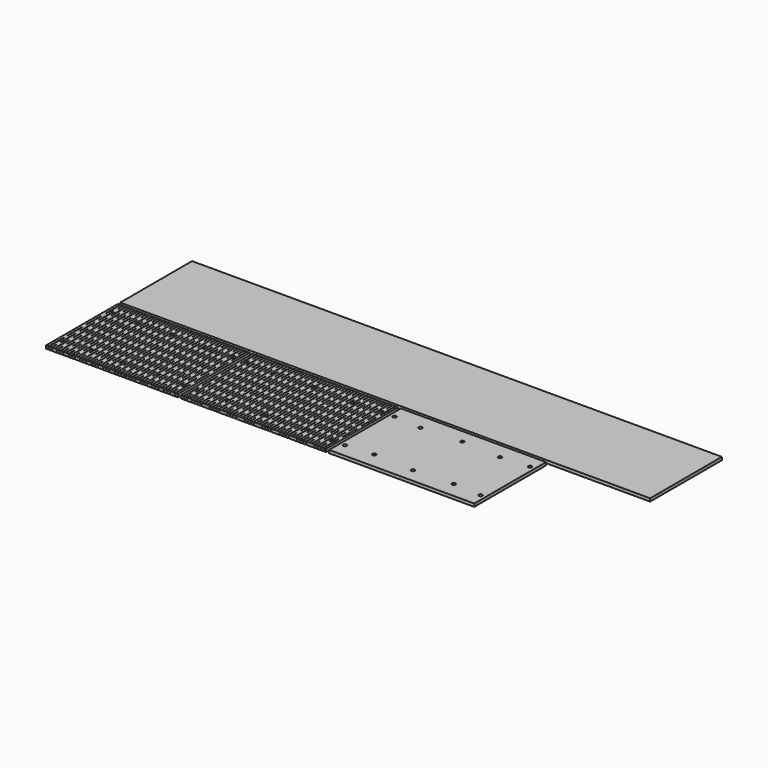
from build123d import *

# Parameters (mm, degrees)
F0_W     = 132.3
F0_H     = 90
F1_DEPTH = 3
F0_W_2   = 531.5
F0_W_3   = 145.6
F2_W     = 0.4
F2_H     = 18.75
F2_H_2   = 6.875
F3_DEPTH = 25
F4_W     = 0.4
F4_H     = 18.75
F4_H_2   = 6.875
F5_DEPTH = 25
F6_D     = 3.5
F6_2_D   = 3.5
F6_3_D   = 3.5
F8_D     = 3.5
F8_2_D   = 3.5
F8_3_D   = 3.5


with BuildPart() as f1:
    # F0 (on Top) → F1 (new body)
    with BuildSketch(Plane.XY):
        with Locations((66.15, -138)):
            Rectangle(F0_W, F0_H)
    extrude(amount=F1_DEPTH)

    # F4 (on face) → F5 (cut)
    with BuildSketch(Plane.XY.offset(3)):
        with Locations((2.7, -173.625)):
            Rectangle(F4_W, F4_H)
        with Locations((5.6, -179.5625)):
            Rectangle(F4_W, F4_H_2)
        with Locations((5.6, -161.75)):
            Rectangle(F4_W, F4_H)
        with Locations((2.7, -149.875)):
            Rectangle(F4_W, F4_H)
        with Locations((5.6, -138)):
            Rectangle(F4_W, F4_H)
        with Locations((2.7, -126.125)):
            Rectangle(F4_W, F4_H)
        with Locations((5.6, -114.25)):
            Rectangle(F4_W, F4_H)
        with Locations((2.7, -102.375)):
            Rectangle(F4_W, F4_H)
        with Locations((5.6, -96.4375)):
            Rectangle(F4_W, F4_H_2)
        with Locations((8.47, -173.625)):
            Rectangle(F4_W, F4_H)
        with Locations((11.37, -179.5625)):
            Rectangle(F4_W, F4_H_2)
        with Locations((11.37, -161.75)):
            Rectangle(F4_W, F4_H)
        with Locations((8.47, -149.875)):
            Rectangle(F4_W, F4_H)
        with Locations((11.37, -138)):
            Rectangle(F4_W, F4_H)
        with Locations((8.47, -126.125)):
            Rectangle(F4_W, F4_H)
        with Locations((11.37, -114.25)):
            Rectangle(F4_W, F4_H)
        with Locations((8.47, -102.375)):
            Rectangle(F4_W, F4_H)
        with Locations((11.37, -96.4375)):
            Rectangle(F4_W, F4_H_2)
        with Locations((14.24, -173.625)):
            Rectangle(F4_W, F4_H)
        with Locations((17.14, -179.5625)):
            Rectangle(F4_W, F4_H_2)
        with Locations((17.14, -161.75)):
            Rectangle(F4_W, F4_H)
        with Locations((14.24, -149.875)):
            Rectangle(F4_W, F4_H)
        with Locations((17.14, -138)):
            Rectangle(F4_W, F4_H)
        with Locations((14.24, -126.125)):
            Rectangle(F4_W, F4_H)
        with Locations((17.14, -114.25)):
            Rectangle(F4_W, F4_H)
        with Locations((14.24, -102.375)):
            Rectangle(F4_W, F4_H)
        with Locations((17.14, -96.4375)):
            Rectangle(F4_W, F4_H_2)
        with Locations((20.01, -173.625)):
            Rectangle(F4_W, F4_H)
        with Locations((22.91, -179.5625)):
            Rectangle(F4_W, F4_H_2)
        with Locations((22.91, -161.75)):
            Rectangle(F4_W, F4_H)
        with Locations((20.01, -149.875)):
            Rectangle(F4_W, F4_H)
        with Locations((22.91, -138)):
            Rectangle(F4_W, F4_H)
        with Locations((20.01, -126.125)):
            Rectangle(F4_W, F4_H)
        with Locations((22.91, -114.25)):
            Rectangle(F4_W, F4_H)
        with Locations((20.01, -102.375)):
            Rectangle(F4_W, F4_H)
        with Locations((22.91, -96.4375)):
            Rectangle(F4_W, F4_H_2)
        with Locations((25.78, -173.625)):
            Rectangle(F4_W, F4_H)
        with Locations((28.68, -179.5625)):
            Rectangle(F4_W, F4_H_2)
        with Locations((28.68, -161.75)):
            Rectangle(F4_W, F4_H)
        with Locations((25.78, -149.875)):
            Rectangle(F4_W, F4_H)
        with Locations((28.68, -138)):
            Rectangle(F4_W, F4_H)
        with Locations((25.78, -126.125)):
            Rectangle(F4_W, F4_H)
        with Locations((28.68, -114.25)):
            Rectangle(F4_W, F4_H)
        with Locations((25.78, -102.375)):
            Rectangle(F4_W, F4_H)
        with Locations((28.68, -96.4375)):
            Rectangle(F4_W, F4_H_2)
        with Locations((31.55, -173.625)):
            Rectangle(F4_W, F4_H)
        with Locations((34.45, -179.5625)):
            Rectangle(F4_W, F4_H_2)
        with Locations((34.45, -161.75)):
            Rectangle(F4_W, F4_H)
        with Locations((31.55, -149.875)):
            Rectangle(F4_W, F4_H)
        with Locations((34.45, -138)):
            Rectangle(F4_W, F4_H)
        with Locations((31.55, -126.125)):
            Rectangle(F4_W, F4_H)
        with Locations((34.45, -114.25)):
            Rectangle(F4_W, F4_H)
        with Locations((31.55, -102.375)):
            Rectangle(F4_W, F4_H)
        with Locations((34.45, -96.4375)):
            Rectangle(F4_W, F4_H_2)
        with Locations((37.32, -173.625)):
            Rectangle(F4_W, F4_H)
        with Locations((40.22, -179.5625)):
            Rectangle(F4_W, F4_H_2)
        with Locations((40.22, -161.75)):
            Rectangle(F4_W, F4_H)
        with Locations((37.32, -149.875)):
            Rectangle(F4_W, F4_H)
        with Locations((40.22, -138)):
            Rectangle(F4_W, F4_H)
        with Locations((37.32, -126.125)):
            Rectangle(F4_W, F4_H)
        with Locations((40.22, -114.25)):
            Rectangle(F4_W, F4_H)
        with Locations((37.32, -102.375)):
            Rectangle(F4_W, F4_H)
        with Locations((40.22, -96.4375)):
            Rectangle(F4_W, F4_H_2)
        with Locations((43.09, -173.625)):
            Rectangle(F4_W, F4_H)
        with Locations((45.99, -179.5625)):
            Rectangle(F4_W, F4_H_2)
        with Locations((45.99, -161.75)):
            Rectangle(F4_W, F4_H)
        with Locations((43.09, -149.875)):
            Rectangle(F4_W, F4_H)
        with Locations((45.99, -138)):
            Rectangle(F4_W, F4_H)
        with Locations((43.09, -126.125)):
            Rectangle(F4_W, F4_H)
        with Locations((45.99, -114.25)):
            Rectangle(F4_W, F4_H)
        with Locations((43.09, -102.375)):
            Rectangle(F4_W, F4_H)
        with Locations((45.99, -96.4375)):
            Rectangle(F4_W, F4_H_2)
        with Locations((48.86, -173.625)):
            Rectangle(F4_W, F4_H)
        with Locations((51.76, -179.5625)):
            Rectangle(F4_W, F4_H_2)
        with Locations((51.76, -161.75)):
            Rectangle(F4_W, F4_H)
        with Locations((48.86, -149.875)):
            Rectangle(F4_W, F4_H)
        with Locations((51.76, -138)):
            Rectangle(F4_W, F4_H)
        with Locations((48.86, -126.125)):
            Rectangle(F4_W, F4_H)
        with Locations((51.76, -114.25)):
            Rectangle(F4_W, F4_H)
        with Locations((48.86, -102.375)):
            Rectangle(F4_W, F4_H)
        with Locations((51.76, -96.4375)):
            Rectangle(F4_W, F4_H_2)
        with Locations((54.63, -173.625)):
            Rectangle(F4_W, F4_H)
        with Locations((57.53, -179.5625)):
            Rectangle(F4_W, F4_H_2)
        with Locations((57.53, -161.75)):
            Rectangle(F4_W, F4_H)
        with Locations((54.63, -149.875)):
            Rectangle(F4_W, F4_H)
        with Locations((57.53, -138)):
            Rectangle(F4_W, F4_H)
        with Locations((54.63, -126.125)):
            Rectangle(F4_W, F4_H)
        with Locations((57.53, -114.25)):
            Rectangle(F4_W, F4_H)
        with Locations((54.63, -102.375)):
            Rectangle(F4_W, F4_H)
        with Locations((57.53, -96.4375)):
            Rectangle(F4_W, F4_H_2)
        with Locations((60.4, -173.625)):
            Rectangle(F4_W, F4_H)
        with Locations((63.3, -179.5625)):
            Rectangle(F4_W, F4_H_2)
        with Locations((63.3, -161.75)):
            Rectangle(F4_W, F4_H)
        with Locations((60.4, -149.875)):
            Rectangle(F4_W, F4_H)
        with Locations((63.3, -138)):
            Rectangle(F4_W, F4_H)
        with Locations((60.4, -126.125)):
            Rectangle(F4_W, F4_H)
        with Locations((63.3, -114.25)):
            Rectangle(F4_W, F4_H)
        with Locations((60.4, -102.375)):
            Rectangle(F4_W, F4_H)
        with Locations((63.3, -96.4375)):
            Rectangle(F4_W, F4_H_2)
        with Locations((66.17, -173.625)):
            Rectangle(F4_W, F4_H)
        with Locations((69.07, -179.5625)):
            Rectangle(F4_W, F4_H_2)
        with Locations((69.07, -161.75)):
            Rectangle(F4_W, F4_H)
        with Locations((66.17, -149.875)):
            Rectangle(F4_W, F4_H)
        with Locations((69.07, -138)):
            Rectangle(F4_W, F4_H)
        with Locations((66.17, -126.125)):
            Rectangle(F4_W, F4_H)
        with Locations((69.07, -114.25)):
            Rectangle(F4_W, F4_H)
        with Locations((66.17, -102.375)):
            Rectangle(F4_W, F4_H)
        with Locations((69.07, -96.4375)):
            Rectangle(F4_W, F4_H_2)
        with Locations((71.94, -173.625)):
            Rectangle(F4_W, F4_H)
        with Locations((74.84, -179.5625)):
            Rectangle(F4_W, F4_H_2)
        with Locations((74.84, -161.75)):
            Rectangle(F4_W, F4_H)
        with Locations((71.94, -149.875)):
            Rectangle(F4_W, F4_H)
        with Locations((74.84, -138)):
            Rectangle(F4_W, F4_H)
        with Locations((71.94, -126.125)):
            Rectangle(F4_W, F4_H)
        with Locations((74.84, -114.25)):
            Rectangle(F4_W, F4_H)
        with Locations((71.94, -102.375)):
            Rectangle(F4_W, F4_H)
        with Locations((74.84, -96.4375)):
            Rectangle(F4_W, F4_H_2)
        with Locations((77.71, -173.625)):
            Rectangle(F4_W, F4_H)
        with Locations((80.61, -179.5625)):
            Rectangle(F4_W, F4_H_2)
        with Locations((80.61, -161.75)):
            Rectangle(F4_W, F4_H)
        with Locations((77.71, -149.875)):
            Rectangle(F4_W, F4_H)
        with Locations((80.61, -138)):
            Rectangle(F4_W, F4_H)
        with Locations((77.71, -126.125)):
            Rectangle(F4_W, F4_H)
        with Locations((80.61, -114.25)):
            Rectangle(F4_W, F4_H)
        with Locations((77.71, -102.375)):
            Rectangle(F4_W, F4_H)
        with Locations((80.61, -96.4375)):
            Rectangle(F4_W, F4_H_2)
        with Locations((83.48, -173.625)):
            Rectangle(F4_W, F4_H)
        with Locations((86.38, -179.5625)):
            Rectangle(F4_W, F4_H_2)
        with Locations((86.38, -161.75)):
            Rectangle(F4_W, F4_H)
        with Locations((83.48, -149.875)):
            Rectangle(F4_W, F4_H)
        with Locations((86.38, -138)):
            Rectangle(F4_W, F4_H)
        with Locations((83.48, -126.125)):
            Rectangle(F4_W, F4_H)
        with Locations((86.38, -114.25)):
            Rectangle(F4_W, F4_H)
        with Locations((83.48, -102.375)):
            Rectangle(F4_W, F4_H)
        with Locations((86.38, -96.4375)):
            Rectangle(F4_W, F4_H_2)
        with Locations((89.25, -173.625)):
            Rectangle(F4_W, F4_H)
        with Locations((92.15, -179.5625)):
            Rectangle(F4_W, F4_H_2)
        with Locations((92.15, -161.75)):
            Rectangle(F4_W, F4_H)
        with Locations((89.25, -149.875)):
            Rectangle(F4_W, F4_H)
        with Locations((92.15, -138)):
            Rectangle(F4_W, F4_H)
        with Locations((89.25, -126.125)):
            Rectangle(F4_W, F4_H)
        with Locations((92.15, -114.25)):
            Rectangle(F4_W, F4_H)
        with Locations((89.25, -102.375)):
            Rectangle(F4_W, F4_H)
        with Locations((92.15, -96.4375)):
            Rectangle(F4_W, F4_H_2)
        with Locations((95.02, -173.625)):
            Rectangle(F4_W, F4_H)
        with Locations((97.92, -179.5625)):
            Rectangle(F4_W, F4_H_2)
        with Locations((97.92, -161.75)):
            Rectangle(F4_W, F4_H)
        with Locations((95.02, -149.875)):
            Rectangle(F4_W, F4_H)
        with Locations((97.92, -138)):
            Rectangle(F4_W, F4_H)
        with Locations((95.02, -126.125)):
            Rectangle(F4_W, F4_H)
        with Locations((97.92, -114.25)):
            Rectangle(F4_W, F4_H)
        with Locations((95.02, -102.375)):
            Rectangle(F4_W, F4_H)
        with Locations((97.92, -96.4375)):
            Rectangle(F4_W, F4_H_2)
        with Locations((100.79, -173.625)):
            Rectangle(F4_W, F4_H)
        with Locations((103.69, -179.5625)):
            Rectangle(F4_W, F4_H_2)
        with Locations((103.69, -161.75)):
            Rectangle(F4_W, F4_H)
        with Locations((100.79, -149.875)):
            Rectangle(F4_W, F4_H)
        with Locations((103.69, -138)):
            Rectangle(F4_W, F4_H)
        with Locations((100.79, -126.125)):
            Rectangle(F4_W, F4_H)
        with Locations((103.69, -114.25)):
            Rectangle(F4_W, F4_H)
        with Locations((100.79, -102.375)):
            Rectangle(F4_W, F4_H)
        with Locations((103.69, -96.4375)):
            Rectangle(F4_W, F4_H_2)
        with Locations((106.56, -173.625)):
            Rectangle(F4_W, F4_H)
        with Locations((109.46, -179.5625)):
            Rectangle(F4_W, F4_H_2)
        with Locations((109.46, -161.75)):
            Rectangle(F4_W, F4_H)
        with Locations((106.56, -149.875)):
            Rectangle(F4_W, F4_H)
        with Locations((109.46, -138)):
            Rectangle(F4_W, F4_H)
        with Locations((106.56, -126.125)):
            Rectangle(F4_W, F4_H)
        with Locations((109.46, -114.25)):
            Rectangle(F4_W, F4_H)
        with Locations((106.56, -102.375)):
            Rectangle(F4_W, F4_H)
        with Locations((109.46, -96.4375)):
            Rectangle(F4_W, F4_H_2)
        with Locations((112.33, -173.625)):
            Rectangle(F4_W, F4_H)
        with Locations((115.23, -179.5625)):
            Rectangle(F4_W, F4_H_2)
        with Locations((115.23, -161.75)):
            Rectangle(F4_W, F4_H)
        with Locations((112.33, -149.875)):
            Rectangle(F4_W, F4_H)
        with Locations((115.23, -138)):
            Rectangle(F4_W, F4_H)
        with Locations((112.33, -126.125)):
            Rectangle(F4_W, F4_H)
        with Locations((115.23, -114.25)):
            Rectangle(F4_W, F4_H)
        with Locations((112.33, -102.375)):
            Rectangle(F4_W, F4_H)
        with Locations((115.23, -96.4375)):
            Rectangle(F4_W, F4_H_2)
        with Locations((118.1, -173.625)):
            Rectangle(F4_W, F4_H)
        with Locations((121, -179.5625)):
            Rectangle(F4_W, F4_H_2)
        with Locations((121, -161.75)):
            Rectangle(F4_W, F4_H)
        with Locations((118.1, -149.875)):
            Rectangle(F4_W, F4_H)
        with Locations((121, -138)):
            Rectangle(F4_W, F4_H)
        with Locations((118.1, -126.125)):
            Rectangle(F4_W, F4_H)
        with Locations((121, -114.25)):
            Rectangle(F4_W, F4_H)
        with Locations((118.1, -102.375)):
            Rectangle(F4_W, F4_H)
        with Locations((121, -96.4375)):
            Rectangle(F4_W, F4_H_2)
        with Locations((123.87, -173.625)):
            Rectangle(F4_W, F4_H)
        with Locations((126.77, -179.5625)):
            Rectangle(F4_W, F4_H_2)
        with Locations((126.77, -161.75)):
            Rectangle(F4_W, F4_H)
        with Locations((123.87, -149.875)):
            Rectangle(F4_W, F4_H)
        with Locations((126.77, -138)):
            Rectangle(F4_W, F4_H)
        with Locations((123.87, -126.125)):
            Rectangle(F4_W, F4_H)
        with Locations((126.77, -114.25)):
            Rectangle(F4_W, F4_H)
        with Locations((123.87, -102.375)):
            Rectangle(F4_W, F4_H)
        with Locations((126.77, -96.4375)):
            Rectangle(F4_W, F4_H_2)
        with Locations((129.64, -173.625)):
            Rectangle(F4_W, F4_H)
        with Locations((132.54, -179.5625)):
            Rectangle(F4_W, F4_H_2)
        with Locations((132.54, -161.75)):
            Rectangle(F4_W, F4_H)
        with Locations((129.64, -149.875)):
            Rectangle(F4_W, F4_H)
        with Locations((132.54, -138)):
            Rectangle(F4_W, F4_H)
        with Locations((129.64, -126.125)):
            Rectangle(F4_W, F4_H)
        with Locations((132.54, -114.25)):
            Rectangle(F4_W, F4_H)
        with Locations((129.64, -102.375)):
            Rectangle(F4_W, F4_H)
        with Locations((132.54, -96.4375)):
            Rectangle(F4_W, F4_H_2)
    extrude(amount=-F5_DEPTH, mode=Mode.SUBTRACT)

    # F6 (through all)
    with Locations(Plane(origin=(0, 0, 0), x_dir=(1, 0, 0), z_dir=(0, 0, -1))):
        with Locations((32.85, 109), (99.45, 109), (32.85, 167), (99.45, 167), (168.65, 109), (168.65, 167), (248.55, 109), (248.55, 167), (316.25, 109), (396.15, 109), (396.15, 167), (316.25, 167)):
            Hole(F6_D / 2)

    # F8 (through all)
    with Locations(Plane.XY.offset(3)):
        with Locations((4.9, -107), (4.9, -169), (127.4, -107), (127.4, -169), (140.2, -107), (140.2, -169), (276, -169), (276, -107), (288.8, -107), (288.8, -169), (424.6, -107), (424.6, -169), (66.15, -107), (66.15, -169), (208.1, -107), (208.1, -169), (356.7, -107), (356.7, -169)):
            Hole(F8_D / 2)


with BuildPart() as f1b:
    # F0 (on Top) → F1, piece 2 (new body)
    with BuildSketch(Plane.XY):
        with Locations((265.75, -45)):
            Rectangle(F0_W_2, F0_H)
    extrude(amount=F1_DEPTH)


with BuildPart() as f1c:
    # F0 (on Top) → F1, piece 3 (new body)
    with BuildSketch(Plane.XY):
        with Locations((208.1, -138)):
            Rectangle(F0_W_3, F0_H)
    extrude(amount=F1_DEPTH)

    # F2 (on face) → F3 (cut)
    with BuildSketch(Plane.XY.offset(3)):
        with Locations((138, -173.625)):
            Rectangle(F2_W, F2_H)
        with Locations((140.9, -179.5625)):
            Rectangle(F2_W, F2_H_2)
        with Locations((140.9, -161.75)):
            Rectangle(F2_W, F2_H)
        with Locations((138, -149.875)):
            Rectangle(F2_W, F2_H)
        with Locations((140.9, -138)):
            Rectangle(F2_W, F2_H)
        with Locations((138, -126.125)):
            Rectangle(F2_W, F2_H)
        with Locations((140.9, -114.25)):
            Rectangle(F2_W, F2_H)
        with Locations((138, -102.375)):
            Rectangle(F2_W, F2_H)
        with Locations((140.9, -96.4375)):
            Rectangle(F2_W, F2_H_2)
        with Locations((146.75, -96.4375)):
            Rectangle(F2_W, F2_H_2)
        with Locations((146.75, -161.75)):
            Rectangle(F2_W, F2_H)
        with Locations((146.75, -114.25)):
            Rectangle(F2_W, F2_H)
        with Locations((143.85, -149.875)):
            Rectangle(F2_W, F2_H)
        with Locations((146.75, -138)):
            Rectangle(F2_W, F2_H)
        with Locations((143.85, -173.625)):
            Rectangle(F2_W, F2_H)
        with Locations((146.75, -179.5625)):
            Rectangle(F2_W, F2_H_2)
        with Locations((143.85, -126.125)):
            Rectangle(F2_W, F2_H)
        with Locations((143.85, -102.375)):
            Rectangle(F2_W, F2_H)
        with Locations((152.6, -96.4375)):
            Rectangle(F2_W, F2_H_2)
        with Locations((152.6, -161.75)):
            Rectangle(F2_W, F2_H)
        with Locations((152.6, -114.25)):
            Rectangle(F2_W, F2_H)
        with Locations((149.7, -149.875)):
            Rectangle(F2_W, F2_H)
        with Locations((152.6, -138)):
            Rectangle(F2_W, F2_H)
        with Locations((149.7, -173.625)):
            Rectangle(F2_W, F2_H)
        with Locations((152.6, -179.5625)):
            Rectangle(F2_W, F2_H_2)
        with Locations((149.7, -126.125)):
            Rectangle(F2_W, F2_H)
        with Locations((149.7, -102.375)):
            Rectangle(F2_W, F2_H)
        with Locations((158.45, -96.4375)):
            Rectangle(F2_W, F2_H_2)
        with Locations((158.45, -161.75)):
            Rectangle(F2_W, F2_H)
        with Locations((158.45, -114.25)):
            Rectangle(F2_W, F2_H)
        with Locations((155.55, -149.875)):
            Rectangle(F2_W, F2_H)
        with Locations((158.45, -138)):
            Rectangle(F2_W, F2_H)
        with Locations((155.55, -173.625)):
            Rectangle(F2_W, F2_H)
        with Locations((158.45, -179.5625)):
            Rectangle(F2_W, F2_H_2)
        with Locations((155.55, -126.125)):
            Rectangle(F2_W, F2_H)
        with Locations((155.55, -102.375)):
            Rectangle(F2_W, F2_H)
        with Locations((164.3, -96.4375)):
            Rectangle(F2_W, F2_H_2)
        with Locations((164.3, -161.75)):
            Rectangle(F2_W, F2_H)
        with Locations((164.3, -114.25)):
            Rectangle(F2_W, F2_H)
        with Locations((161.4, -149.875)):
            Rectangle(F2_W, F2_H)
        with Locations((164.3, -138)):
            Rectangle(F2_W, F2_H)
        with Locations((161.4, -173.625)):
            Rectangle(F2_W, F2_H)
        with Locations((164.3, -179.5625)):
            Rectangle(F2_W, F2_H_2)
        with Locations((161.4, -126.125)):
            Rectangle(F2_W, F2_H)
        with Locations((161.4, -102.375)):
            Rectangle(F2_W, F2_H)
        with Locations((170.15, -96.4375)):
            Rectangle(F2_W, F2_H_2)
        with Locations((170.15, -161.75)):
            Rectangle(F2_W, F2_H)
        with Locations((170.15, -114.25)):
            Rectangle(F2_W, F2_H)
        with Locations((167.25, -149.875)):
            Rectangle(F2_W, F2_H)
        with Locations((170.15, -138)):
            Rectangle(F2_W, F2_H)
        with Locations((167.25, -173.625)):
            Rectangle(F2_W, F2_H)
        with Locations((170.15, -179.5625)):
            Rectangle(F2_W, F2_H_2)
        with Locations((167.25, -126.125)):
            Rectangle(F2_W, F2_H)
        with Locations((167.25, -102.375)):
            Rectangle(F2_W, F2_H)
        with Locations((176, -96.4375)):
            Rectangle(F2_W, F2_H_2)
        with Locations((176, -161.75)):
            Rectangle(F2_W, F2_H)
        with Locations((176, -114.25)):
            Rectangle(F2_W, F2_H)
        with Locations((173.1, -149.875)):
            Rectangle(F2_W, F2_H)
        with Locations((176, -138)):
            Rectangle(F2_W, F2_H)
        with Locations((173.1, -173.625)):
            Rectangle(F2_W, F2_H)
        with Locations((176, -179.5625)):
            Rectangle(F2_W, F2_H_2)
        with Locations((173.1, -126.125)):
            Rectangle(F2_W, F2_H)
        with Locations((173.1, -102.375)):
            Rectangle(F2_W, F2_H)
        with Locations((181.85, -96.4375)):
            Rectangle(F2_W, F2_H_2)
        with Locations((181.85, -161.75)):
            Rectangle(F2_W, F2_H)
        with Locations((181.85, -114.25)):
            Rectangle(F2_W, F2_H)
        with Locations((178.95, -149.875)):
            Rectangle(F2_W, F2_H)
        with Locations((181.85, -138)):
            Rectangle(F2_W, F2_H)
        with Locations((178.95, -173.625)):
            Rectangle(F2_W, F2_H)
        with Locations((181.85, -179.5625)):
            Rectangle(F2_W, F2_H_2)
        with Locations((178.95, -126.125)):
            Rectangle(F2_W, F2_H)
        with Locations((178.95, -102.375)):
            Rectangle(F2_W, F2_H)
        with Locations((187.7, -96.4375)):
            Rectangle(F2_W, F2_H_2)
        with Locations((187.7, -161.75)):
            Rectangle(F2_W, F2_H)
        with Locations((187.7, -114.25)):
            Rectangle(F2_W, F2_H)
        with Locations((184.8, -149.875)):
            Rectangle(F2_W, F2_H)
        with Locations((187.7, -138)):
            Rectangle(F2_W, F2_H)
        with Locations((184.8, -173.625)):
            Rectangle(F2_W, F2_H)
        with Locations((187.7, -179.5625)):
            Rectangle(F2_W, F2_H_2)
        with Locations((184.8, -126.125)):
            Rectangle(F2_W, F2_H)
        with Locations((184.8, -102.375)):
            Rectangle(F2_W, F2_H)
        with Locations((193.55, -96.4375)):
            Rectangle(F2_W, F2_H_2)
        with Locations((193.55, -161.75)):
            Rectangle(F2_W, F2_H)
        with Locations((193.55, -114.25)):
            Rectangle(F2_W, F2_H)
        with Locations((190.65, -149.875)):
            Rectangle(F2_W, F2_H)
        with Locations((193.55, -138)):
            Rectangle(F2_W, F2_H)
        with Locations((190.65, -173.625)):
            Rectangle(F2_W, F2_H)
        with Locations((193.55, -179.5625)):
            Rectangle(F2_W, F2_H_2)
        with Locations((190.65, -126.125)):
            Rectangle(F2_W, F2_H)
        with Locations((190.65, -102.375)):
            Rectangle(F2_W, F2_H)
        with Locations((199.4, -96.4375)):
            Rectangle(F2_W, F2_H_2)
        with Locations((199.4, -161.75)):
            Rectangle(F2_W, F2_H)
        with Locations((199.4, -114.25)):
            Rectangle(F2_W, F2_H)
        with Locations((196.5, -149.875)):
            Rectangle(F2_W, F2_H)
        with Locations((199.4, -138)):
            Rectangle(F2_W, F2_H)
        with Locations((196.5, -173.625)):
            Rectangle(F2_W, F2_H)
        with Locations((199.4, -179.5625)):
            Rectangle(F2_W, F2_H_2)
        with Locations((196.5, -126.125)):
            Rectangle(F2_W, F2_H)
        with Locations((196.5, -102.375)):
            Rectangle(F2_W, F2_H)
        with Locations((205.25, -96.4375)):
            Rectangle(F2_W, F2_H_2)
        with Locations((205.25, -161.75)):
            Rectangle(F2_W, F2_H)
        with Locations((205.25, -114.25)):
            Rectangle(F2_W, F2_H)
        with Locations((202.35, -149.875)):
            Rectangle(F2_W, F2_H)
        with Locations((205.25, -138)):
            Rectangle(F2_W, F2_H)
        with Locations((202.35, -173.625)):
            Rectangle(F2_W, F2_H)
        with Locations((205.25, -179.5625)):
            Rectangle(F2_W, F2_H_2)
        with Locations((202.35, -126.125)):
            Rectangle(F2_W, F2_H)
        with Locations((202.35, -102.375)):
            Rectangle(F2_W, F2_H)
        with Locations((211.1, -96.4375)):
            Rectangle(F2_W, F2_H_2)
        with Locations((211.1, -161.75)):
            Rectangle(F2_W, F2_H)
        with Locations((211.1, -114.25)):
            Rectangle(F2_W, F2_H)
        with Locations((208.2, -149.875)):
            Rectangle(F2_W, F2_H)
        with Locations((211.1, -138)):
            Rectangle(F2_W, F2_H)
        with Locations((208.2, -173.625)):
            Rectangle(F2_W, F2_H)
        with Locations((211.1, -179.5625)):
            Rectangle(F2_W, F2_H_2)
        with Locations((208.2, -126.125)):
            Rectangle(F2_W, F2_H)
        with Locations((208.2, -102.375)):
            Rectangle(F2_W, F2_H)
        with Locations((216.95, -96.4375)):
            Rectangle(F2_W, F2_H_2)
        with Locations((216.95, -161.75)):
            Rectangle(F2_W, F2_H)
        with Locations((216.95, -114.25)):
            Rectangle(F2_W, F2_H)
        with Locations((214.05, -149.875)):
            Rectangle(F2_W, F2_H)
        with Locations((216.95, -138)):
            Rectangle(F2_W, F2_H)
        with Locations((214.05, -173.625)):
            Rectangle(F2_W, F2_H)
        with Locations((216.95, -179.5625)):
            Rectangle(F2_W, F2_H_2)
        with Locations((214.05, -126.125)):
            Rectangle(F2_W, F2_H)
        with Locations((214.05, -102.375)):
            Rectangle(F2_W, F2_H)
        with Locations((222.8, -96.4375)):
            Rectangle(F2_W, F2_H_2)
        with Locations((222.8, -161.75)):
            Rectangle(F2_W, F2_H)
        with Locations((222.8, -114.25)):
            Rectangle(F2_W, F2_H)
        with Locations((219.9, -149.875)):
            Rectangle(F2_W, F2_H)
        with Locations((222.8, -138)):
            Rectangle(F2_W, F2_H)
        with Locations((219.9, -173.625)):
            Rectangle(F2_W, F2_H)
        with Locations((222.8, -179.5625)):
            Rectangle(F2_W, F2_H_2)
        with Locations((219.9, -126.125)):
            Rectangle(F2_W, F2_H)
        with Locations((219.9, -102.375)):
            Rectangle(F2_W, F2_H)
        with Locations((228.65, -96.4375)):
            Rectangle(F2_W, F2_H_2)
        with Locations((228.65, -161.75)):
            Rectangle(F2_W, F2_H)
        with Locations((228.65, -114.25)):
            Rectangle(F2_W, F2_H)
        with Locations((225.75, -149.875)):
            Rectangle(F2_W, F2_H)
        with Locations((228.65, -138)):
            Rectangle(F2_W, F2_H)
        with Locations((225.75, -173.625)):
            Rectangle(F2_W, F2_H)
        with Locations((228.65, -179.5625)):
            Rectangle(F2_W, F2_H_2)
        with Locations((225.75, -126.125)):
            Rectangle(F2_W, F2_H)
        with Locations((225.75, -102.375)):
            Rectangle(F2_W, F2_H)
        with Locations((234.5, -96.4375)):
            Rectangle(F2_W, F2_H_2)
        with Locations((234.5, -161.75)):
            Rectangle(F2_W, F2_H)
        with Locations((234.5, -114.25)):
            Rectangle(F2_W, F2_H)
        with Locations((231.6, -149.875)):
            Rectangle(F2_W, F2_H)
        with Locations((234.5, -138)):
            Rectangle(F2_W, F2_H)
        with Locations((231.6, -173.625)):
            Rectangle(F2_W, F2_H)
        with Locations((234.5, -179.5625)):
            Rectangle(F2_W, F2_H_2)
        with Locations((231.6, -126.125)):
            Rectangle(F2_W, F2_H)
        with Locations((231.6, -102.375)):
            Rectangle(F2_W, F2_H)
        with Locations((240.35, -96.4375)):
            Rectangle(F2_W, F2_H_2)
        with Locations((240.35, -161.75)):
            Rectangle(F2_W, F2_H)
        with Locations((240.35, -114.25)):
            Rectangle(F2_W, F2_H)
        with Locations((237.45, -149.875)):
            Rectangle(F2_W, F2_H)
        with Locations((240.35, -138)):
            Rectangle(F2_W, F2_H)
        with Locations((237.45, -173.625)):
            Rectangle(F2_W, F2_H)
        with Locations((240.35, -179.5625)):
            Rectangle(F2_W, F2_H_2)
        with Locations((237.45, -126.125)):
            Rectangle(F2_W, F2_H)
        with Locations((237.45, -102.375)):
            Rectangle(F2_W, F2_H)
        with Locations((246.2, -96.4375)):
            Rectangle(F2_W, F2_H_2)
        with Locations((246.2, -161.75)):
            Rectangle(F2_W, F2_H)
        with Locations((246.2, -114.25)):
            Rectangle(F2_W, F2_H)
        with Locations((243.3, -149.875)):
            Rectangle(F2_W, F2_H)
        with Locations((246.2, -138)):
            Rectangle(F2_W, F2_H)
        with Locations((243.3, -173.625)):
            Rectangle(F2_W, F2_H)
        with Locations((246.2, -179.5625)):
            Rectangle(F2_W, F2_H_2)
        with Locations((243.3, -126.125)):
            Rectangle(F2_W, F2_H)
        with Locations((243.3, -102.375)):
            Rectangle(F2_W, F2_H)
        with Locations((252.05, -96.4375)):
            Rectangle(F2_W, F2_H_2)
        with Locations((252.05, -161.75)):
            Rectangle(F2_W, F2_H)
        with Locations((252.05, -114.25)):
            Rectangle(F2_W, F2_H)
        with Locations((249.15, -149.875)):
            Rectangle(F2_W, F2_H)
        with Locations((252.05, -138)):
            Rectangle(F2_W, F2_H)
        with Locations((249.15, -173.625)):
            Rectangle(F2_W, F2_H)
        with Locations((252.05, -179.5625)):
            Rectangle(F2_W, F2_H_2)
        with Locations((249.15, -126.125)):
            Rectangle(F2_W, F2_H)
        with Locations((249.15, -102.375)):
            Rectangle(F2_W, F2_H)
        with Locations((257.9, -96.4375)):
            Rectangle(F2_W, F2_H_2)
        with Locations((257.9, -161.75)):
            Rectangle(F2_W, F2_H)
        with Locations((257.9, -114.25)):
            Rectangle(F2_W, F2_H)
        with Locations((255, -149.875)):
            Rectangle(F2_W, F2_H)
        with Locations((257.9, -138)):
            Rectangle(F2_W, F2_H)
        with Locations((255, -173.625)):
            Rectangle(F2_W, F2_H)
        with Locations((257.9, -179.5625)):
            Rectangle(F2_W, F2_H_2)
        with Locations((255, -126.125)):
            Rectangle(F2_W, F2_H)
        with Locations((255, -102.375)):
            Rectangle(F2_W, F2_H)
        with Locations((263.75, -96.4375)):
            Rectangle(F2_W, F2_H_2)
        with Locations((263.75, -161.75)):
            Rectangle(F2_W, F2_H)
        with Locations((263.75, -114.25)):
            Rectangle(F2_W, F2_H)
        with Locations((260.85, -149.875)):
            Rectangle(F2_W, F2_H)
        with Locations((263.75, -138)):
            Rectangle(F2_W, F2_H)
        with Locations((260.85, -173.625)):
            Rectangle(F2_W, F2_H)
        with Locations((263.75, -179.5625)):
            Rectangle(F2_W, F2_H_2)
        with Locations((260.85, -126.125)):
            Rectangle(F2_W, F2_H)
        with Locations((260.85, -102.375)):
            Rectangle(F2_W, F2_H)
        with Locations((269.6, -96.4375)):
            Rectangle(F2_W, F2_H_2)
        with Locations((269.6, -161.75)):
            Rectangle(F2_W, F2_H)
        with Locations((269.6, -114.25)):
            Rectangle(F2_W, F2_H)
        with Locations((266.7, -149.875)):
            Rectangle(F2_W, F2_H)
        with Locations((269.6, -138)):
            Rectangle(F2_W, F2_H)
        with Locations((266.7, -173.625)):
            Rectangle(F2_W, F2_H)
        with Locations((269.6, -179.5625)):
            Rectangle(F2_W, F2_H_2)
        with Locations((266.7, -126.125)):
            Rectangle(F2_W, F2_H)
        with Locations((266.7, -102.375)):
            Rectangle(F2_W, F2_H)
        with Locations((275.45, -96.4375)):
            Rectangle(F2_W, F2_H_2)
        with Locations((275.45, -161.75)):
            Rectangle(F2_W, F2_H)
        with Locations((275.45, -114.25)):
            Rectangle(F2_W, F2_H)
        with Locations((272.55, -149.875)):
            Rectangle(F2_W, F2_H)
        with Locations((275.45, -138)):
            Rectangle(F2_W, F2_H)
        with Locations((272.55, -173.625)):
            Rectangle(F2_W, F2_H)
        with Locations((275.45, -179.5625)):
            Rectangle(F2_W, F2_H_2)
        with Locations((272.55, -126.125)):
            Rectangle(F2_W, F2_H)
        with Locations((272.55, -102.375)):
            Rectangle(F2_W, F2_H)
        with Locations((281.3, -96.4375)):
            Rectangle(F2_W, F2_H_2)
        with Locations((281.3, -161.75)):
            Rectangle(F2_W, F2_H)
        with Locations((281.3, -114.25)):
            Rectangle(F2_W, F2_H)
        with Locations((278.4, -149.875)):
            Rectangle(F2_W, F2_H)
        with Locations((281.3, -138)):
            Rectangle(F2_W, F2_H)
        with Locations((278.4, -173.625)):
            Rectangle(F2_W, F2_H)
        with Locations((281.3, -179.5625)):
            Rectangle(F2_W, F2_H_2)
        with Locations((278.4, -126.125)):
            Rectangle(F2_W, F2_H)
        with Locations((278.4, -102.375)):
            Rectangle(F2_W, F2_H)
    extrude(amount=-F3_DEPTH, mode=Mode.SUBTRACT)

    # F6#2 (through all)
    with Locations(Plane(origin=(0, 0, 0), x_dir=(1, 0, 0), z_dir=(0, 0, -1))):
        with Locations((32.85, 109), (99.45, 109), (32.85, 167), (99.45, 167), (168.65, 109), (168.65, 167), (248.55, 109), (248.55, 167), (316.25, 109), (396.15, 109), (396.15, 167), (316.25, 167)):
            Hole(F6_2_D / 2)

    # F8#2 (through all)
    with Locations(Plane.XY.offset(3)):
        with Locations((4.9, -107), (4.9, -169), (127.4, -107), (127.4, -169), (140.2, -107), (140.2, -169), (276, -169), (276, -107), (288.8, -107), (288.8, -169), (424.6, -107), (424.6, -169), (66.15, -107), (66.15, -169), (208.1, -107), (208.1, -169), (356.7, -107), (356.7, -169)):
            Hole(F8_2_D / 2)


with BuildPart() as f1d:
    # F0 (on Top) → F1, piece 4 (new body)
    with BuildSketch(Plane.XY):
        with Locations((356.7, -138)):
            Rectangle(F0_W_3, F0_H)
    extrude(amount=F1_DEPTH)

    # F6#3 (through all)
    with Locations(Plane(origin=(0, 0, 0), x_dir=(1, 0, 0), z_dir=(0, 0, -1))):
        with Locations((32.85, 109), (99.45, 109), (32.85, 167), (99.45, 167), (168.65, 109), (168.65, 167), (248.55, 109), (248.55, 167), (316.25, 109), (396.15, 109), (396.15, 167), (316.25, 167)):
            Hole(F6_3_D / 2)

    # F8#3 (through all)
    with Locations(Plane.XY.offset(3)):
        with Locations((4.9, -107), (4.9, -169), (127.4, -107), (127.4, -169), (140.2, -107), (140.2, -169), (276, -169), (276, -107), (288.8, -107), (288.8, -169), (424.6, -107), (424.6, -169), (66.15, -107), (66.15, -169), (208.1, -107), (208.1, -169), (356.7, -107), (356.7, -169)):
            Hole(F8_3_D / 2)


solid = Compound([f1.part, f1b.part, f1c.part, f1d.part])
